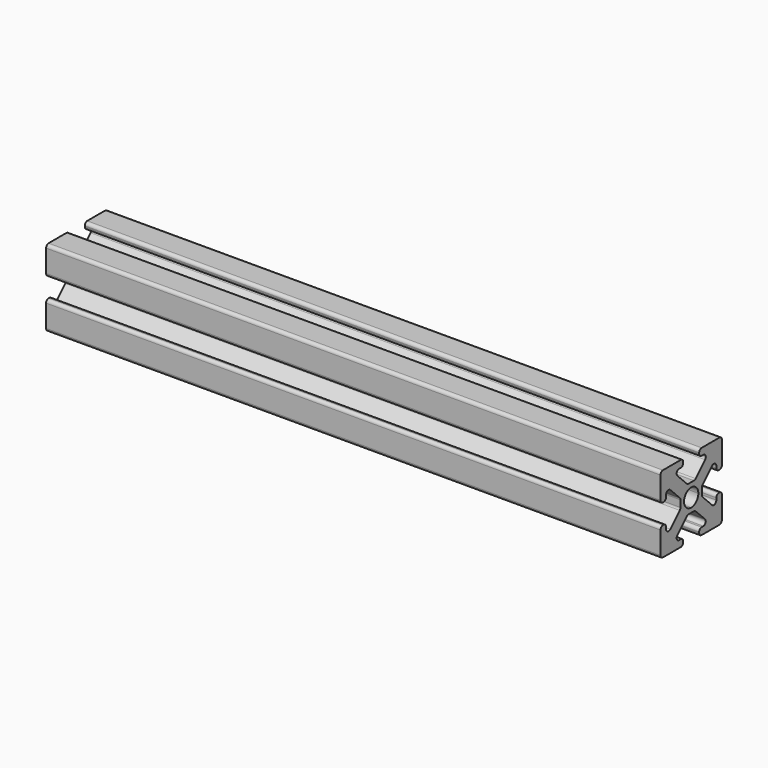
from build123d import *

# Parameters (mm, degrees)
F0_W             = 12.5
F0_H             = 25
F1_DEPTH         = 100
F2_W             = 2.28
F2_H             = 3.25
F3_DEPTH         = 200
F3_COPIES_COUNT  = 2
F3_COPIES_ANGLE  = 90
F3_COPIES1_COUNT = 2
F3_COPIES1_ANGLE = 270
F5_R             = 1
F7_R             = 2.5374832391
F8_DEPTH         = 200


# Not quite as in the source:
# - a pattern or mirror of a feature is missing from the dataset's text; its kind, count and spacing are read off the source's solid


with BuildPart() as f1:
    # F0 (on Right) → F1 (new body, symmetric)
    with BuildSketch(Plane.YZ):
        with Locations((-6.25, 12.5)):
            Rectangle(F0_W, F0_H)
        Polygon((0, 0), (12.5, 0), (12.5, 9.25), (10.22, 9.25), (10.22, 5.155), (4.38, 5.155), (4.38, 9.25), (4.38, 10.995), (4.38, 14.005), (4.38, 15.75), (4.38, 19.845), (10.22, 19.845), (10.22, 15.75), (12.5, 15.75), (12.5, 25), (0, 25), align=None)
        Polygon((10.22, 5.155), (6.125, 9.25), (4.38, 9.25), (4.38, 5.155), align=None)
        Polygon((4.38, 9.25), (6.125, 9.25), (4.38, 10.995), align=None)
        Polygon((4.38, 14.005), (6.125, 15.75), (4.38, 15.75), align=None)
        Polygon((4.38, 15.75), (6.125, 15.75), (10.22, 19.845), (4.38, 19.845), align=None)
    extrude(amount=F1_DEPTH, both=True)

    # F2 (on face) → F3 (cut, through all)
    with BuildSketch(Plane(origin=(-100, 0, 0), x_dir=(0, -1, 0), z_dir=(-1, 0, 0))):
        with Locations((11.36, 10.875)):
            Rectangle(F2_W, F2_H)
        with BuildLine():
            Line((0, 15.0374832391), (0, 9.9625167609))
            ThreePointArc((0, 9.9625167609), (1.7942716055, 10.7057283945), (2.5374832391, 12.5))
            ThreePointArc((2.5374832391, 12.5), (1.7942716055, 14.2942716055), (0, 15.0374832391))
        make_face()
        with Locations((11.36, 14.125)):
            Rectangle(F2_W, F2_H)
        Polygon((10.22, 5.155), (10.22, 9.25), (6.125, 9.25), align=None)
        Polygon((6.125, 9.25), (10.22, 9.25), (10.22, 12.5), (10.22, 15.75), (6.125, 15.75), (4.38, 14.005), (4.38, 10.995), align=None)
        Polygon((6.125, 15.75), (10.22, 15.75), (10.22, 19.845), align=None)
    f3 = extrude(amount=-F3_DEPTH, mode=Mode.SUBTRACT)

    # F3_copies: F3 ×2 about axis
    f3_copies_axis = Axis((0, 0, 12.5), (1, 0, 0))
    for i in range(1, F3_COPIES_COUNT):
        add(f3.rotate(f3_copies_axis, i * F3_COPIES_ANGLE / (F3_COPIES_COUNT - 1)), mode=Mode.SUBTRACT)

    # F3_copies1: F3 ×2 about axis
    f3_copies1_axis = Axis((0, 0, 12.5), (1, 0, 0))
    for i in range(1, F3_COPIES1_COUNT):
        add(f3.rotate(f3_copies1_axis, i * F3_COPIES1_ANGLE / (F3_COPIES1_COUNT - 1)), mode=Mode.SUBTRACT)

    # F5
    f5_edges = [f1.edges().sort_by_distance(p)[0] for p in [
        (0, -4.38, 14.005),
        (0, -4.38, 10.995),
        (0, -10.22, 19.845),
        (0, -10.22, 15.75),
        (0, -12.5, 15.75),
        (0, -12.5, 9.25),
        (0, -10.22, 9.25),
        (0, -10.22, 5.155),
        (0, 12.5, 25),
        (0, -12.5, 25),
        (0, -12.5, 0),
        (0, 12.5, 0),
        (0, 10.22, 19.845),
        (0, 10.22, 15.75),
        (0, 4.38, 14.005),
        (0, 4.38, 10.995),
        (0, 10.22, 5.155),
        (0, 10.22, 9.25),
        (0, 12.5, 9.25),
        (0, 3.25, 0),
        (0, 3.25, 2.28),
        (0, 7.345, 2.28),
        (0, 1.505, 8.12),
        (0, -1.505, 8.12),
        (0, -7.345, 2.28),
        (0, -3.25, 2.28),
        (0, -3.25, 0),
        (0, -3.25, 22.72),
        (0, -3.25, 25),
        (0, -7.345, 22.72),
        (0, -1.505, 16.88),
        (0, 1.505, 16.88),
        (0, 7.345, 22.72),
        (0, 3.25, 22.72),
        (0, 3.25, 25),
        (0, 12.5, 15.75),
    ]]
    fillet(f5_edges, radius=F5_R)

    # F7 (on face) → F8 (cut, through all)
    with BuildSketch(Plane(origin=(-100, 0, 0), x_dir=(0, -1, 0), z_dir=(-1, 0, 0))):
        with BuildLine():
            ThreePointArc((0, 9.5939878347), (2.0548609083, 10.4451390917), (2.9060121653, 12.5))
            ThreePointArc((2.9060121653, 12.5), (2.0548609083, 14.5548609083), (0, 15.4060121653))
            ThreePointArc((0, 15.4060121653), (-2.0548609083, 14.5548609083), (-2.9060121653, 12.5))
            ThreePointArc((-2.9060121653, 12.5), (-2.0548609083, 10.4451390917), (0, 9.5939878347))
        make_face()
        with Locations((0, 12.5)):
            Circle(F7_R, mode=Mode.SUBTRACT)
    extrude(amount=-F8_DEPTH, mode=Mode.SUBTRACT)


solid = f1.part
